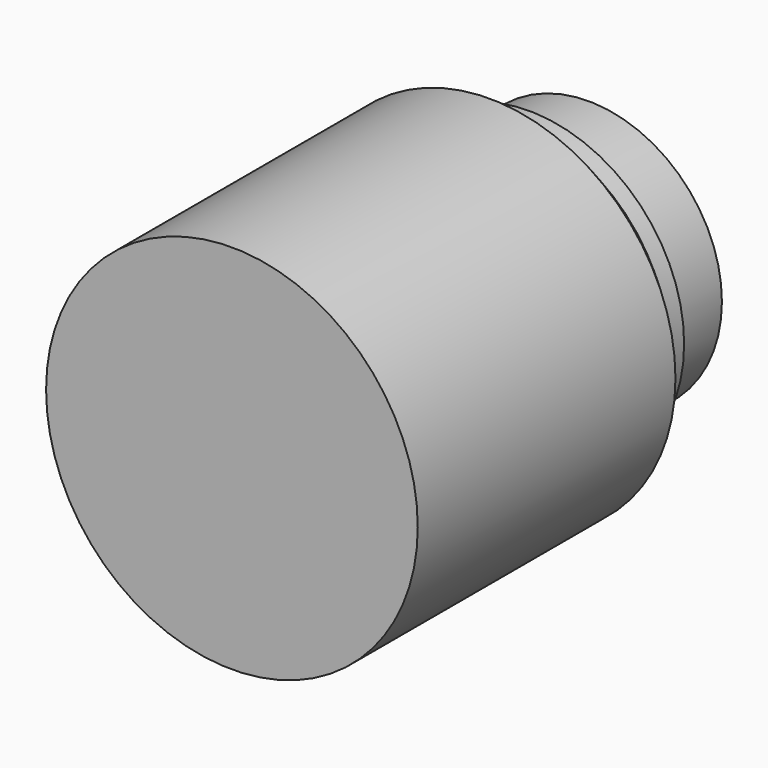
from build123d import *

# Parameters (mm, degrees)
F0_W    = 0.7
F0_H    = 0.6
F2_SIZE = 0.99999


# Not quite as in the source:
# - a fillet or chamfer is up to 0.001 mm smaller than in the source, because OpenCascade refuses the exact size


with BuildPart() as f1:
    # F0 (on Top) → F1 (revolve)
    with BuildSketch(Plane.XY):
        with Locations((4.65, 11.7)):
            Rectangle(F0_W, F0_H)
        Polygon((0, 14.4), (0, 0), (6, 0), (6, 11.4), (5, 11.4), (4.3, 11.4), (4.3, 12), (4.3, 14.4), align=None)
    revolve(axis=Axis((0, 7.2, 0), (0, 1, 0)))

    # F2 (size 1 in the source; OpenCascade refuses exactly that, so slightly less here)
    f2_edges = [f1.edges().sort_by_distance(p)[0] for p in [
        (-6, 11.4, 0),
    ]]
    chamfer(f2_edges, length=F2_SIZE)


solid = f1.part
